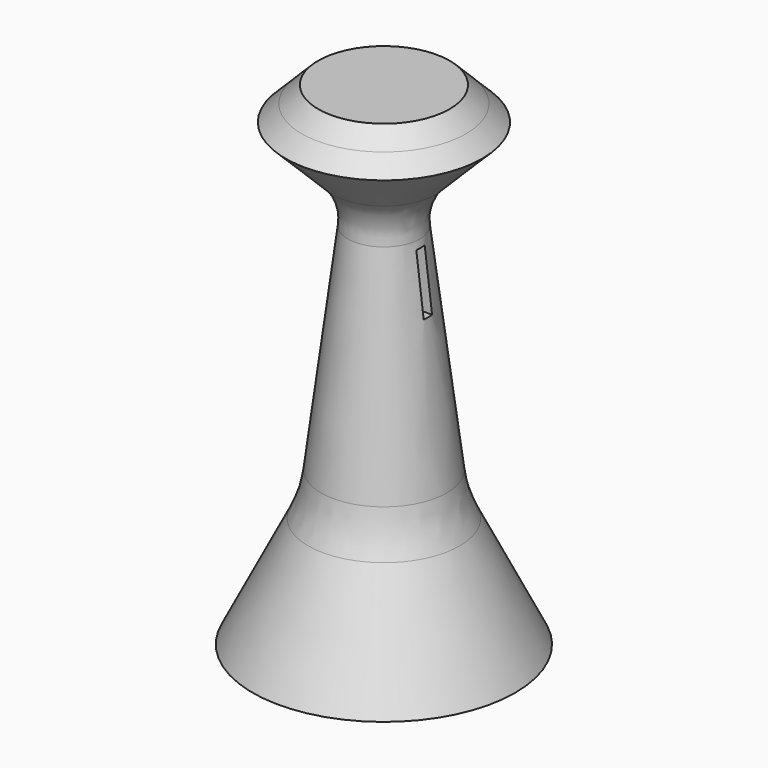
from build123d import *

# Parameters (mm, degrees)
F0_R           = 12.7
F2_R           = 6.35
F3_FACE_R      = 6.35
F5_R           = 3.175
F6_FACE_R      = 3.175
F8_R           = 9.525
F10_R          = 12.7
F11_R          = 5.08
F9_FACE_R      = 9.525
F13_R          = 7.9375
F16_R          = 6.35
F14_FACE_R     = 7.9375
F18_W          = 0.508
F18_H          = 5.6896
F19_DEPTH      = 12.7010001
F19_DEPTH_BACK = 25.4
F20_DEPTH      = 1.27


with BuildPart() as f3:
    # F0 (on Top) → F3 section 0
    with BuildSketch(Plane.XY):
        Circle(F0_R)
    # F2 (on offset) → F3 section 1
    with BuildSketch(Plane.XY.offset(12.7)):
        Circle(F2_R)
    loft()

    # F3_face (on face) → F6 section 0
    with BuildSketch(Plane.XY.offset(12.7)):
        Circle(F3_FACE_R)
    # F5 (on offset) → F6 section 1
    with BuildSketch(Plane.XY.offset(38.1)):
        Circle(F5_R)
    loft()

    # F6_face (on face) → F9 section 0
    with BuildSketch(Plane.XY.offset(38.1)):
        Circle(F6_FACE_R)
    # F8 (on offset) → F9 section 1
    with BuildSketch(Plane.XY.offset(44.45)):
        Circle(F8_R)
    loft()

    # F10
    f10_edges = [f3.edges().sort_by_distance(p)[0] for p in [
        (-6.35, 0, 12.7),
    ]]
    fillet(f10_edges, radius=F10_R)

    # F11
    f11_edges = [f3.edges().sort_by_distance(p)[0] for p in [
        (-3.175, 0, 38.1),
    ]]
    fillet(f11_edges, radius=F11_R)

    # F9_face (on face) → F14 section 0
    with BuildSketch(Plane.XY.offset(44.45)):
        Circle(F9_FACE_R)
    # F13 (on offset) → F14 section 1
    with BuildSketch(Plane.XY.offset(46.0375)):
        Circle(F13_R)
    loft()

    # F16 (on offset) → F17 section 0
    with BuildSketch(Plane.XY.offset(47.625)):
        Circle(F16_R)
    # F14_face (on face) → F17 section 1
    with BuildSketch(Plane.XY.offset(46.0375)):
        Circle(F14_FACE_R)
    loft()

    # F18 (on Right) → F19 (cut, two sides)
    with BuildSketch(Plane.YZ) as f19_sk:
        with Locations((0.254, 32.0802)):
            Rectangle(F18_W, F18_H)
        with Locations((-0.254, 32.0802)):
            Rectangle(F18_W, F18_H)
    extrude(amount=-F19_DEPTH, mode=Mode.SUBTRACT)
    extrude(f19_sk.sketch, amount=F19_DEPTH_BACK, mode=Mode.SUBTRACT)

    # F18 (on Right) → F20 (join, symmetric)
    with BuildSketch(Plane.YZ):
        with Locations((0.254, 32.0802)):
            Rectangle(F18_W, F18_H)
        with Locations((-0.254, 32.0802)):
            Rectangle(F18_W, F18_H)
    extrude(amount=F20_DEPTH, both=True)


solid = f3.part
